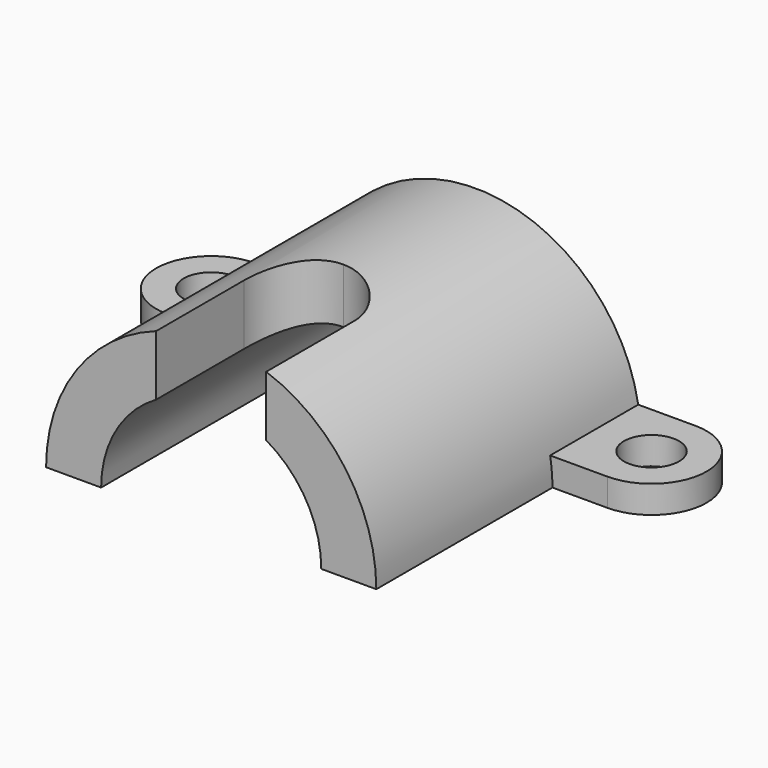
from build123d import *

# Parameters (mm, degrees)
F2_DEPTH  = 60
F4_DEPTH  = 5
F5_R      = 5
F6_DEPTH  = 5
F8_DEPTH  = 30.0010001
F9_R      = 20
F10_DEPTH = 60.0010001


# Not quite as in the source:
# - a pattern or mirror of a feature is missing from the dataset's text; its kind, count and spacing are read off the source's solid


with BuildPart() as f2:
    # F1 (on Front) → F2 (new body)
    with BuildSketch(Plane.XZ):
        with BuildLine():
            Line((-30, 0), (30, 0))
            ThreePointArc((30, 0), (0, 30), (-30, 0))
        make_face()
    extrude(amount=-F2_DEPTH)

    # F3 (on Top) → F4 (join)
    with BuildSketch(Plane.XY):
        with BuildLine():
            ThreePointArc((-40, 60), (-50, 50), (-40, 40))
            Line((-40, 40), (40, 40))
            ThreePointArc((40, 40), (50, 50), (40, 60))
            Line((40, 60), (-40, 60))
        make_face()
    extrude(amount=F4_DEPTH)

    # F5 (on Top) → F6 (cut, through all)
    with BuildSketch(Plane.XY):
        with Locations((-40, 50)):
            Circle(F5_R)
    f6 = extrude(amount=F6_DEPTH, mode=Mode.SUBTRACT)

    # F6_copies: F6 across plane
    add(f6.mirror(Plane(origin=(0, 0, 0), x_dir=(0, 0, 1), z_dir=(1, 0, 0))), mode=Mode.SUBTRACT)

    # F7 (on Top) → F8 (cut, through all)
    with BuildSketch(Plane.XY):
        with BuildLine():
            Line((-10, 20), (-10, 0))
            Line((-10, 0), (0, 0))
            Line((0, 0), (0, 30))
            ThreePointArc((0, 30), (-7.0710678119, 27.0710678119), (-10, 20))
        make_face()
        with BuildLine():
            Line((0, 30), (0, 0))
            Line((0, 0), (10, 0))
            Line((10, 0), (10, 20))
            ThreePointArc((10, 20), (7.0710678119, 27.0710678119), (0, 30))
        make_face()
    extrude(amount=F8_DEPTH, mode=Mode.SUBTRACT)

    # F9 (on face) → F10 (cut, through all)
    with BuildSketch(Plane.XZ):
        Circle(F9_R)
    extrude(amount=-F10_DEPTH, mode=Mode.SUBTRACT)


solid = f2.part
